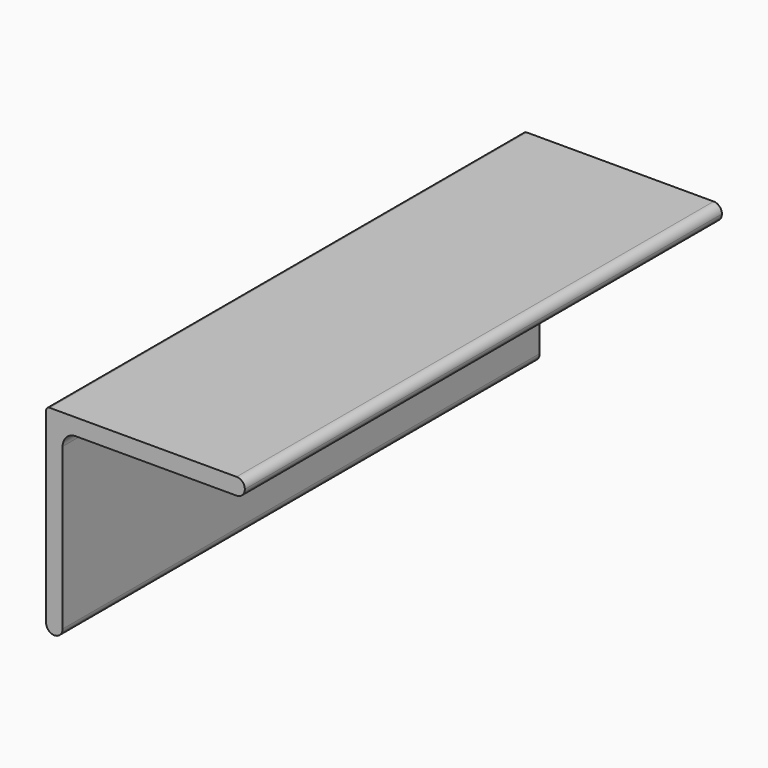
from build123d import *

# Parameters (mm, degrees)
F1_DEPTH = 114.3
F2_R     = 5.08
F3_R     = 3.17499
F4_R     = 1.397


# Not quite as in the source:
# - a fillet or chamfer is up to 0.001 mm smaller than in the source, because OpenCascade refuses the exact size


with BuildPart() as f1:
    # F0 (on Front) → F1 (new body, symmetric)
    with BuildSketch(Plane.XZ):
        Polygon((76.2, 0), (0, 0), (0, -76.2), (6.35, -76.2), (6.35, -6.35), (76.2, -6.35), align=None)
    extrude(amount=F1_DEPTH, both=True)

    # F2
    f2_edges = [f1.edges().sort_by_distance(p)[0] for p in [
        (6.35, 0, -6.35),
    ]]
    fillet(f2_edges, radius=F2_R)

    # F3 (radius 3.175 in the source; OpenCascade refuses exactly that, so slightly less here)
    f3_edges = [f1.edges().sort_by_distance(p)[0] for p in [
        (76.2, 0, -6.35),
        (76.2, 0, 0),
        (0, 0, -76.2),
        (6.35, 0, -76.2),
    ]]
    fillet(f3_edges, radius=F3_R)

    # F4
    f4_edges = [f1.edges().sort_by_distance(p)[0] for p in [
        (0, 0, 0),
    ]]
    fillet(f4_edges, radius=F4_R)


solid = f1.part
